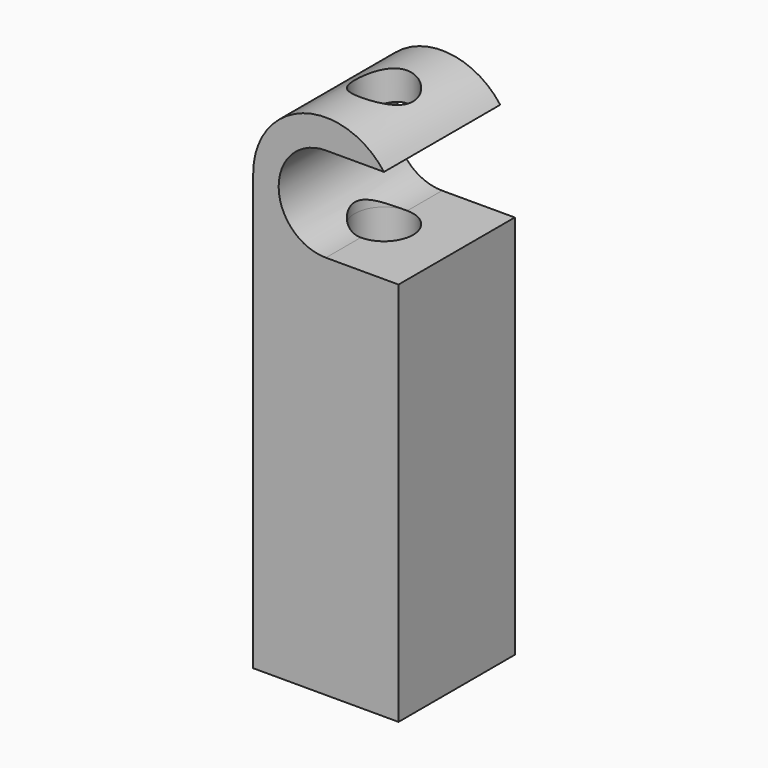
from build123d import *

# Parameters (mm, degrees)
F1_DEPTH      = 10
F1_DEPTH_BACK = 10
F3_DEPTH      = 20
F4_R          = 4
F5_DEPTH      = 40
F5_DEPTH_BACK = 18.0000001001
F7_D          = 3.5


with BuildPart() as f1:
    # F0 (on Front) → F1 (new body, two sides)
    with BuildSketch(Plane.XZ) as f1_sk:
        with BuildLine():
            ThreePointArc((10, 60), (0, 70), (-10, 60))
            Line((-10, 60), (-10, 0))
            Line((-10, 0), (10, 0))
            Line((10, 0), (10, 60))
        make_face()
    extrude(amount=F1_DEPTH)
    extrude(f1_sk.sketch, amount=-F1_DEPTH_BACK)

    # F2 (on face) → F3 (cut, through all)
    with BuildSketch(Plane(origin=(0, 10, 0), x_dir=(-1, 0, 0), z_dir=(0, 1, 0))):
        with BuildLine():
            Line((-10, 53), (0, 53))
            ThreePointArc((0, 53), (6.5, 59.5), (0, 66))
            Line((0, 66), (-8, 66))
            ThreePointArc((-8, 66), (-9.4868329805, 63.1622776602), (-10, 60))
            Line((-10, 60), (-10, 53))
        make_face()
    extrude(amount=-F3_DEPTH, mode=Mode.SUBTRACT)

    # F4 (on face) → F5 (cut, two sides)
    with BuildSketch(Plane.XY.offset(53)) as f5_sk:
        Circle(F4_R)
    extrude(amount=-F5_DEPTH, mode=Mode.SUBTRACT)
    extrude(f5_sk.sketch, amount=F5_DEPTH_BACK, mode=Mode.SUBTRACT)

    # F7 (through all)
    with Locations(Plane.XY.offset(13)):
        with Locations((0, 0)):
            Hole(F7_D / 2)


solid = f1.part
